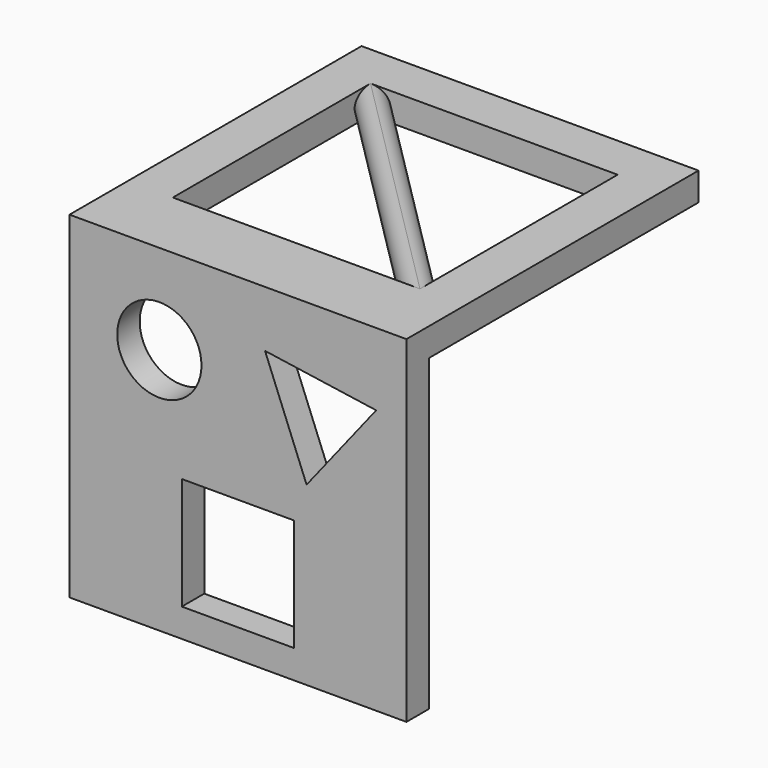
from build123d import *

# Parameters (mm, degrees)
F0_W     = 76.2
F0_H     = 76.2
F0_W_2   = 25.4
F0_H_2   = 25.4
F0_R     = 9.525
F1_DEPTH = 6.35
F2_W     = 76.2
F2_H     = 76.2
F3_DEPTH = 6.35
F4_DEPTH = 6.35
F5_R     = 3.17499


# Not quite as in the source:
# - a fillet or chamfer is up to 0.001 mm smaller than in the source, because OpenCascade refuses the exact size


with BuildPart() as f1:
    # F0 (on Front) → F1 (new body)
    with BuildSketch(Plane.XZ):
        Rectangle(F0_W, F0_H)
        with Locations((0, -18.9619082958)):
            Rectangle(F0_W_2, F0_H_2, mode=Mode.SUBTRACT)
        with Locations((-17.78, 17.78)):
            Circle(F0_R, mode=Mode.SUBTRACT)
        Polygon((15.5130978999, 1.7698944463), (6.1174177746, 25.3682247894), (31.2520114013, 21.7059572922), align=None, mode=Mode.SUBTRACT)
    extrude(amount=-F1_DEPTH)

    # F2 (on face) → F3 (join)
    with BuildSketch(Plane.XY.offset(38.1)):
        with Locations((0, 44.45)):
            Rectangle(F2_W, F2_H)
        Polygon((-27.94, 67.8998719395), (-27.94, 72.39), (-23.4498719395, 72.39), (27.94, 72.39), (27.94, 21.0001280605), (27.94, 16.51), (23.4498719395, 16.51), (-27.94, 16.51), align=None, mode=Mode.SUBTRACT)
    extrude(amount=-F3_DEPTH)

    # F2 (on face) → F4 (join)
    with BuildSketch(Plane.XY.offset(38.1)):
        Polygon((-23.4498719395, 72.39), (-27.94, 72.39), (-27.94, 67.8998719395), (23.4498719395, 16.51), (27.94, 16.51), (27.94, 21.0001280605), align=None)
    extrude(amount=-F4_DEPTH)

    # F5 (radius 3.175 in the source; OpenCascade refuses exactly that, so slightly less here)
    f5_edges = [f1.edges().sort_by_distance(p)[0] for p in [
        (2.245064, 46.695064, 38.1),
        (-2.245064, 42.204936, 38.1),
        (-2.245064, 42.204936, 31.75),
        (2.245064, 46.695064, 31.75),
    ]]
    fillet(f5_edges, radius=F5_R)


solid = f1.part
